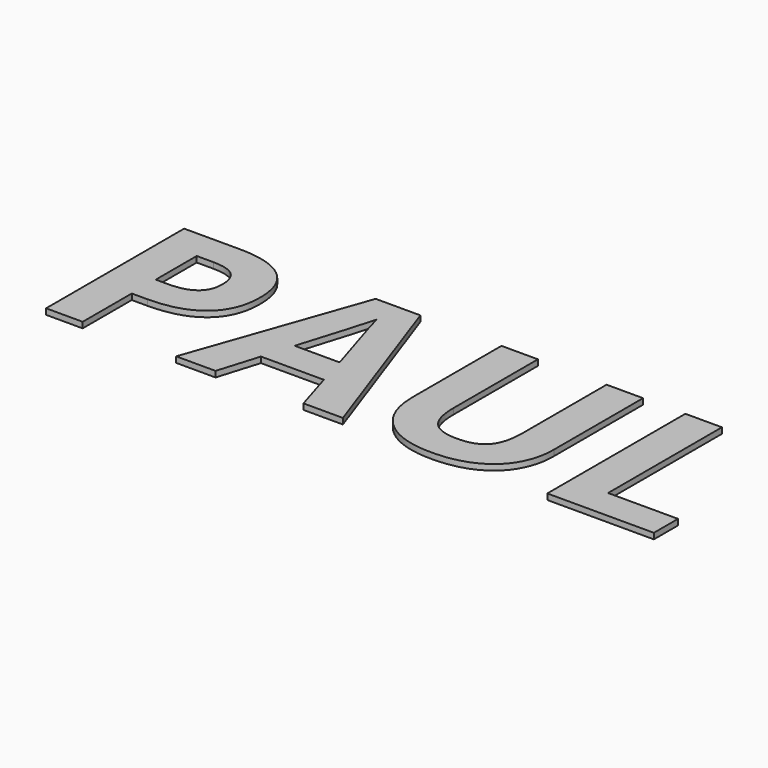
from build123d import *

# Parameters (mm, degrees)
F0_TEXT_SIZE = 41.6666666667
F1_DEPTH     = 1


# Not quite as in the source:
# - Text() gives the source's letters only with a copy of the font that has no kerning and outlines rounded to 1/6400 em; it was checked with that copy


with BuildPart() as f1:
    # F0 (on Top) → F1 (new body)
    with BuildSketch(Plane.XY):
        with Locations((-55.615234375, 0)):
            Text('PAUL', F0_TEXT_SIZE, font='Open Sans', font_style=FontStyle.BOLD, text_align=(TextAlign.LEFT, TextAlign.BOTTOM))
    extrude(amount=F1_DEPTH)


solid = f1.part
